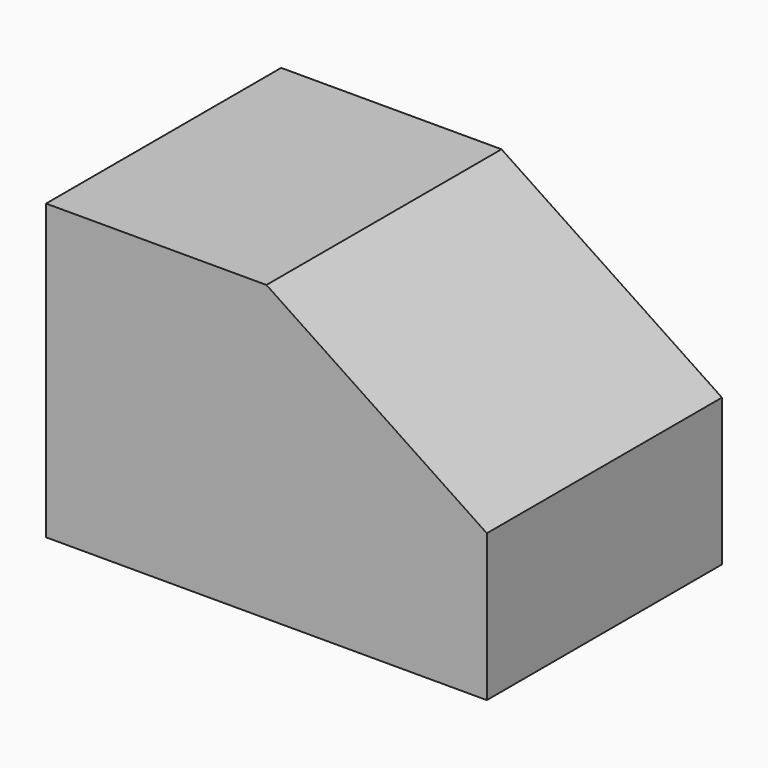
from build123d import *

# Parameters (mm, degrees)
F0_R     = 12.7
F1_DEPTH = 25.4


# Not quite as in the source:
# - the program builds the solid bodies; features that only make, move or delete a surface that nothing else refers to are left out


with BuildPart() as f1:
    # F0 (on Front) → F1 (new body, symmetric)
    with BuildSketch(Plane.XZ):
        Polygon((-38.1, 25.4), (-38.1, -25.4), (38.1, -25.4), (38.1, 0), (0, 25.4), align=None)
        Circle(F0_R, mode=Mode.SUBTRACT)
        Circle(F0_R)
    extrude(amount=F1_DEPTH, both=True)


solid = f1.part
